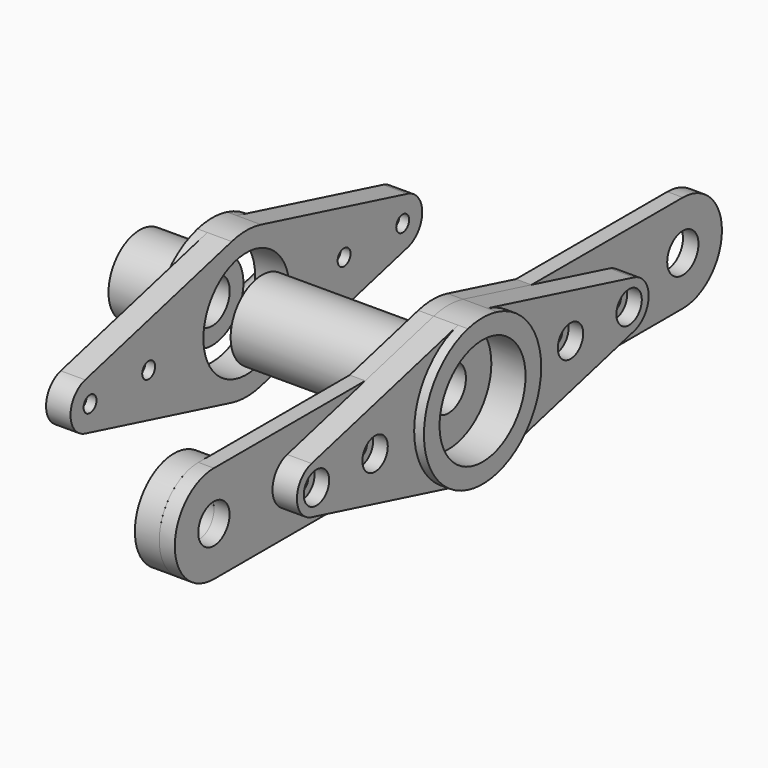
from build123d import *

# Parameters (mm, degrees)
F0_R             = 11
F1_DEPTH         = 7
F2_DEPTH         = 5
F3_R             = 4
F3_R_2           = 4.5
F4_DEPTH         = 3.175
F6_D             = 3.3
F6_DEPTH         = 16
F6_CBORE_D       = 6.5
F6_CBORE_DEPTH   = 3
F6_TIP           = 0.9914200214
F6_2_D           = 3.3
F6_2_DEPTH       = 16
F6_2_CBORE_D     = 6.5
F6_2_CBORE_DEPTH = 3
F6_2_TIP         = 0.9914200214
F7_R             = 8
F7_R_2           = 4.5
F8_DEPTH         = 35
F11_R            = 10
F11_R_2          = 4
F12_DEPTH        = 5
F15_DEPTH        = 25
F16_R            = 1.25
F17_DEPTH        = 25
F19_R            = 8
F19_R_2          = 4.5
F20_DEPTH        = 14.825


# Not quite as in the source:
# - a length typed as a fraction of an inch, garbled in the dataset ("3 / 203.2 mm" for 3/8 in), is restored


with BuildPart() as f1:
    # F0 (on Right) → F1 (new body)
    with BuildSketch(Plane.YZ):
        with BuildLine():
            ThreePointArc((3.75, -14.5236875483), (11.8585412256, -9.1855865354), (15, 0))
            ThreePointArc((15, 0), (11.8585412256, 9.1855865354), (3.75, 14.5236875483))
            ThreePointArc((3.75, 14.5236875483), (0, 15), (-3.75, 14.5236875483))
            ThreePointArc((-3.75, 14.5236875483), (-15, 0), (-3.75, -14.5236875483))
            ThreePointArc((-3.75, -14.5236875483), (0, -15), (3.75, -14.5236875483))
        make_face()
        Circle(F0_R, mode=Mode.SUBTRACT)
    extrude(amount=F1_DEPTH)

    # F0 (on Right) → F2 (join)
    with BuildSketch(Plane.YZ):
        with BuildLine():
            ThreePointArc((-3.75, -14.5236875483), (-15, 0), (-3.75, 14.5236875483))
            Line((-3.75, 14.5236875483), (-41.25, 4.8412291828))
            ThreePointArc((-41.25, 4.8412291828), (-45, 0), (-41.25, -4.8412291828))
            Line((-41.25, -4.8412291828), (-3.75, -14.5236875483))
        make_face()
        with BuildLine():
            ThreePointArc((3.75, 14.5236875483), (11.8585412256, 9.1855865354), (15, 0))
            ThreePointArc((15, 0), (11.8585412256, -9.1855865354), (3.75, -14.5236875483))
            Line((3.75, -14.5236875483), (41.25, -4.8412291828))
            ThreePointArc((41.25, -4.8412291828), (45, 0), (41.25, 4.8412291828))
            Line((41.25, 4.8412291828), (3.75, 14.5236875483))
        make_face()
    extrude(amount=F2_DEPTH)

    # F6
    with Locations(Plane.YZ.offset(5)):
        with Locations((-40, 0), (40, 0), (-25, 0), (25, 0)):
            CounterBoreHole(F6_D / 2, F6_CBORE_D / 2, F6_CBORE_DEPTH, depth=F6_DEPTH)
            with Locations((0, 0, -(F6_DEPTH + F6_TIP / 2))):  # 118° drill point
                Cone(0, F6_D / 2, F6_TIP, mode=Mode.SUBTRACT)


with BuildPart() as f4:
    # F3 (on face) → F4 (new body)
    with BuildSketch(Plane(origin=(0, 0, 0), x_dir=(0, -1, 0), z_dir=(-1, 0, 0))):
        with BuildLine():
            Line((-21.2701665379, -10), (-3.75, -14.5236875483))
            ThreePointArc((-3.75, -14.5236875483), (0, -15), (3.75, -14.5236875483))
            Line((3.75, -14.5236875483), (21.2701665379, -10))
            Line((21.2701665379, -10), (60, -10))
            ThreePointArc((60, -10), (70, 0), (60, 10))
            Line((60, 10), (21.2701665379, 10))
            Line((21.2701665379, 10), (3.75, 14.5236875483))
            ThreePointArc((3.75, 14.5236875483), (0, 15), (-3.75, 14.5236875483))
            Line((-3.75, 14.5236875483), (-21.2701665379, 10))
            Line((-21.2701665379, 10), (-60, 10))
            ThreePointArc((-60, 10), (-70, 0), (-60, -10))
            Line((-60, -10), (-21.2701665379, -10))
        make_face()
        with Locations((-60, 0)):
            Circle(F3_R, mode=Mode.SUBTRACT)
        Circle(F3_R_2, mode=Mode.SUBTRACT)
        with Locations((60, 0)):
            Circle(F3_R, mode=Mode.SUBTRACT)
    extrude(amount=F4_DEPTH)

    # F6#2
    with Locations(Plane.YZ.offset(5)):
        with Locations((-40, 0), (40, 0), (-25, 0), (25, 0)):
            CounterBoreHole(F6_2_D / 2, F6_2_CBORE_D / 2, F6_2_CBORE_DEPTH, depth=F6_2_DEPTH)
            with Locations((0, 0, -(F6_2_DEPTH + F6_2_TIP / 2))):  # 118° drill point
                Cone(0, F6_2_D / 2, F6_2_TIP, mode=Mode.SUBTRACT)


with BuildPart() as f8:
    # F7 (on face) → F8 (new body)
    with BuildSketch(Plane(origin=(-3.175, 0, 0), x_dir=(0, -1, 0), z_dir=(-1, 0, 0))):
        Circle(F7_R)
        Circle(F7_R_2, mode=Mode.SUBTRACT)
    extrude(amount=F8_DEPTH)


with BuildPart() as f12:
    # F11 (on offset) → F12 (new body, through all)
    with BuildSketch(Plane.YZ.offset(-8.175)):
        with Locations((-60, 0)):
            Circle(F11_R)
        with Locations((-60, 0)):
            Circle(F11_R_2, mode=Mode.SUBTRACT)
    extrude(amount=F12_DEPTH)


with BuildPart() as f13_1:
    # F13: instance of F1
    add(f1.part.mirror(Plane(origin=(-20.675, 0, 0), x_dir=(0, -1, 0), z_dir=(1, 0, 0))))

    # F14 (on face) → F15 (join)
    with BuildSketch(Plane(origin=(-46.35, 0, 0), x_dir=(0, -1, 0), z_dir=(-1, 0, 0))):
        Polygon((-20.0660774882, -1.130489487), (-21.5105219326, -6.7247987649), (-11.8280635671, -9.2247987649), (-10.3836191227, -3.630489487), align=None)
    extrude(amount=F15_DEPTH)

    # F16 (on face) → F17 (cut)
    with BuildSketch(Plane(origin=(0, 8.8558413449, 2.286568403), x_dir=(1, 0, 0), z_dir=(0, -0.9682458366, -0.25))):
        with BuildLine():
            ThreePointArc((-50.6, -11.8888888889), (-53.4888888889, -9), (-50.6, -6.1111111111))
            Line((-50.6, -6.1111111111), (-50.6, 4.3424948306))
            Line((-50.6, 4.3424948306), (-79.8189531028, 4.3424948306))
            Line((-79.8189531028, 4.3424948306), (-79.8189531028, -25.2762112579))
            Line((-79.8189531028, -25.2762112579), (-50.6, -25.2762112579))
            Line((-50.6, -25.2762112579), (-50.6, -11.8888888889))
        make_face()
        with Locations((-50.6, -9)):
            Circle(F16_R)
    extrude(amount=-F17_DEPTH, mode=Mode.SUBTRACT)


with BuildPart() as f20:
    # F19 (on offset) → F20 (new body, through all)
    with BuildSketch(Plane.YZ.offset(-63.175)):
        Circle(F19_R)
        Circle(F19_R_2, mode=Mode.SUBTRACT)
    extrude(amount=F20_DEPTH)


solid = Compound([f1.part, f4.part, f8.part, f12.part, f13_1.part, f20.part])
